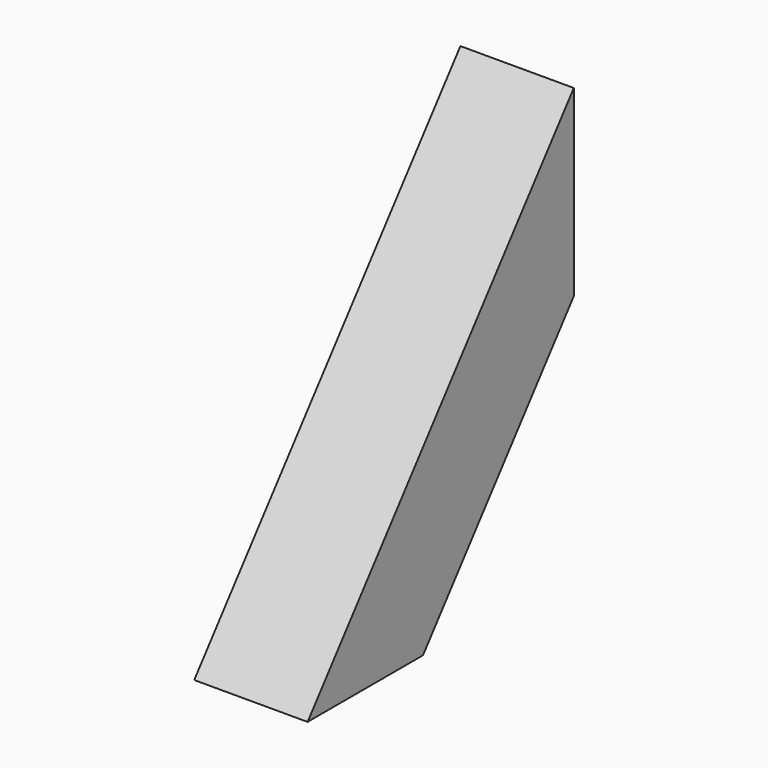
from build123d import *

# Parameters (mm, degrees)
F1_DEPTH      = 7.9375
F4_W          = 7.6985172927
F4_H          = 8.837191388
F5_DEPTH      = 32.041668515
F5_DEPTH_BACK = 25.4


with BuildPart() as f1:
    # F6 (on Right) → F1 (new body, symmetric)
    with BuildSketch(Plane.YZ):
        Polygon((46.5895857938, 59.2058200122), (0, 0), (20.2007462682, 0), (46.5895857938, 33.5348094786), align=None)
    extrude(amount=F1_DEPTH, both=True)

    # F4 (on face) → F5 (cut, two sides)
    with BuildSketch(Plane(origin=(0, 20.9196058881, 26.5845338574), x_dir=(1, 0, 0), z_dir=(0, -0.6184018342, -0.7858620562))) as f5_sk:
        with Locations((0, -11.8702491745)):
            Rectangle(F4_W, F4_H)
    extrude(amount=-F5_DEPTH, mode=Mode.SUBTRACT)
    extrude(f5_sk.sketch, amount=F5_DEPTH_BACK, mode=Mode.SUBTRACT)


solid = f1.part
